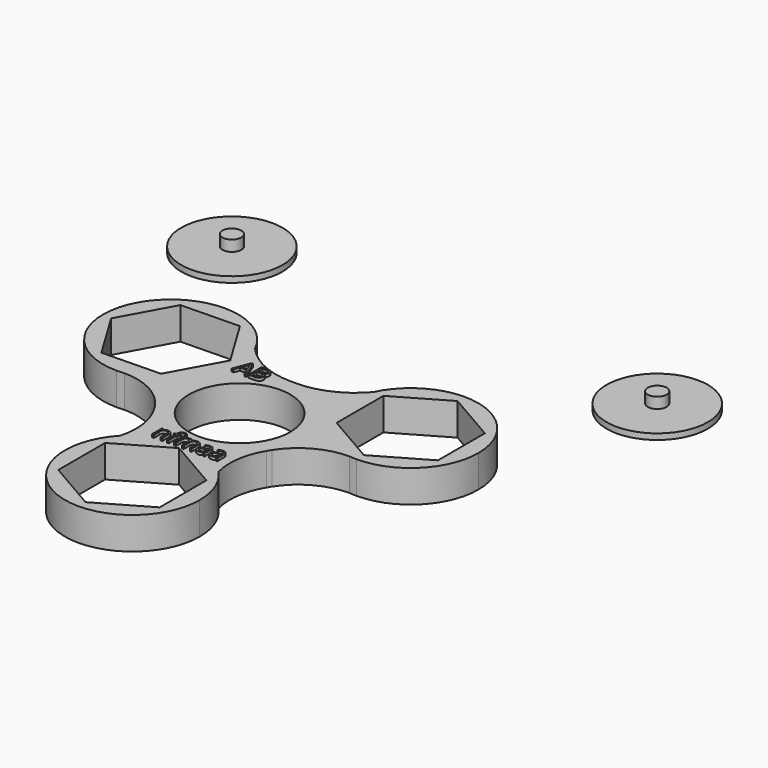
from build123d import *

# Parameters (mm, degrees)
F0_R           = 11.0297341738
F1_DEPTH       = 7.0104
F2_TEXT_SIZE   = 5.0108763389
F2_TEXT_SIZE_2 = 5.0108750454
F3_DEPTH       = 7.62
F4_R           = 2.0485624903
F5_DEPTH       = 3.6322
F4_R_2         = 11.0106906114
F6_DEPTH       = 1.27
F7_DEPTH       = 3.6322
F8_DEPTH       = 1.27


# Not quite as in the source:
# - Text() gives the source's letters only with a copy of the font that has no kerning and outlines rounded to 1/6400 em; it was checked with that copy


with BuildPart() as f1:
    # F0 (on Top) → F1 (new body)
    with BuildSketch(Plane.XY):
        with BuildLine():
            ThreePointArc((12.7688238327, -7.0845952005), (14.1366843581, -3.6590308258), (14.6025460528, 0))
            ThreePointArc((14.6025460528, 0), (10.512006113, 10.1356834356), (0.5321122622, 14.5928478292))
            ThreePointArc((0.5321122622, 14.5928478292), (0.2660161908, 14.5955055395), (0, 14.6025460528))
            ThreePointArc((0, 14.6025460528), (-0.2660161908, 14.5955055395), (-0.5321122622, 14.5928478292))
            ThreePointArc((-0.5321122622, 14.5928478292), (-12.7163913641, 7.1782826567), (-12.7688238327, -7.0845952005))
            ThreePointArc((-12.7688238327, -7.0845952005), (-12.5014299415, -7.5119719558), (-12.2495942672, -7.9486974727))
            ThreePointArc((-12.2495942672, -7.9486974727), (-7.4978531693, -12.5306244488), (-1.2139729432, -14.5519971453))
            ThreePointArc((-1.2139729432, -14.5519971453), (0, -14.50165494), (1.2139729432, -14.5519971453))
            ThreePointArc((1.2139729432, -14.5519971453), (7.4978531693, -12.5306244488), (12.2495942672, -7.9486974727))
            ThreePointArc((12.2495942672, -7.9486974727), (12.5014299415, -7.5119719558), (12.7688238327, -7.0845952005))
        make_face()
        Circle(F0_R, mode=Mode.SUBTRACT)
        with BuildLine():
            ThreePointArc((0.5321122622, 14.5928478292), (10.512006113, 10.1356834356), (14.6025460528, 0))
            ThreePointArc((14.6025460528, 0), (14.1366843581, -3.6590308258), (12.7688238327, -7.0845952005))
            ThreePointArc((12.7688238327, -7.0845952005), (17.81162254, -2.4243097964), (24.4636618418, -0.7218257358))
            ThreePointArc((24.4636618418, -0.7218257358), (13.2399010204, 6.7733722545), (12.8515015084, 20.2641078056))
            ThreePointArc((12.8515015084, 20.2641078056), (7.3157643156, 16.0730868655), (0.5321122622, 14.5928478292))
        make_face()
        with BuildLine():
            ThreePointArc((0, 14.6025460528), (0.2660161908, 14.5955055395), (0.5321122622, 14.5928478292))
            ThreePointArc((0.5321122622, 14.5928478292), (0.2661003171, 14.6001212956), (0, 14.6025460528))
        make_face()
        with BuildLine():
            ThreePointArc((12.2495942672, -7.9486974727), (12.5166680566, -7.5211283718), (12.7688238327, -7.0845952005))
            ThreePointArc((12.7688238327, -7.0845952005), (12.5014299415, -7.5119719558), (12.2495942672, -7.9486974727))
        make_face()
        with BuildLine():
            ThreePointArc((-0.5321122622, 14.5928478292), (-0.2660161908, 14.5955055395), (0, 14.6025460528))
            ThreePointArc((0, 14.6025460528), (-0.2661003171, 14.6001212956), (-0.5321122622, 14.5928478292))
        make_face()
        with BuildLine():
            ThreePointArc((40.8192647261, 13.8948662207), (29.3762925366, 28.2367891894), (12.8515015084, 20.2641078056))
            ThreePointArc((12.8515015084, 20.2641078056), (13.2399010204, 6.7733722545), (24.4636618418, -0.7218257358))
            ThreePointArc((24.4636618418, -0.7218257358), (25.2882595444, -0.7437857189), (26.1101331562, -0.8142653492))
            ThreePointArc((26.1101331562, -0.8142653492), (36.5110598346, 3.4939395422), (40.8192647261, 13.8948662207))
        make_face()
        Polygon((26.1101331562, 26.6333493906), (37.1419831871, 20.2641078056), (37.1419831871, 7.5256246357), (26.1101331562, 1.1563830507), (15.0782831253, 7.5256246357), (15.0782831253, 20.2641078056), align=None, mode=Mode.SUBTRACT)
        with BuildLine():
            ThreePointArc((10.6742573559, -19.1119285094), (10.3201713626, -13.3691904701), (12.2495942672, -7.9486974727))
            ThreePointArc((12.2495942672, -7.9486974727), (7.4978531693, -12.5306244488), (1.2139729432, -14.5519971453))
            ThreePointArc((1.2139729432, -14.5519971453), (6.3663763965, -15.9559164192), (10.6742573559, -19.1119285094))
        make_face()
        with BuildLine():
            ThreePointArc((26.1101331562, -0.8142653492), (25.2882595444, -0.7437857189), (24.4636618418, -0.7218257358))
            ThreePointArc((24.4636618418, -0.7218257358), (25.2856010357, -0.791137263), (26.1101331562, -0.8142653492))
        make_face()
        with BuildLine():
            ThreePointArc((-12.7688238327, -7.0845952005), (-12.7163913641, 7.1782826567), (-0.5321122622, 14.5928478292))
            ThreePointArc((-0.5321122622, 14.5928478292), (-7.3157643157, 16.0730868655), (-12.8515015084, 20.2641078056))
            ThreePointArc((-12.8515015084, 20.2641078056), (-11.7682101874, 17.161025601), (-11.4010015863, 13.8948662207))
            ThreePointArc((-11.4010015863, 13.8948662207), (-15.1425282506, 4.0933258226), (-24.4636618418, -0.7218257358))
            ThreePointArc((-24.4636618418, -0.7218257358), (-17.81162254, -2.4243097964), (-12.7688238327, -7.0845952005))
        make_face()
        with BuildLine():
            ThreePointArc((10.6742573559, -19.1119285094), (6.3663763965, -15.9559164192), (1.2139729432, -14.5519971453))
            ThreePointArc((1.2139729432, -14.5519971453), (0, -14.6025460528), (-1.2139729432, -14.5519971453))
            ThreePointArc((-1.2139729432, -14.5519971453), (-6.3663763965, -15.9559164192), (-10.6742573559, -19.1119285094))
            ThreePointArc((-10.6742573559, -19.1119285094), (-5.4071159221, -42.792818386), (14.6622961142, -29.1639510542))
            ThreePointArc((14.6622961142, -29.1639510542), (13.6288673318, -23.7568351321), (10.6742573559, -19.1119285094))
        make_face()
        Polygon((0, -41.889001257), (-11.02021674, -35.5264761556), (-11.02021674, -22.8014259528), (0, -16.4389008515), (11.02021674, -22.8014259528), (11.02021674, -35.5264761556), align=None, mode=Mode.SUBTRACT)
        with BuildLine():
            ThreePointArc((-12.2495942672, -7.9486974727), (-12.5014299415, -7.5119719558), (-12.7688238327, -7.0845952005))
            ThreePointArc((-12.7688238327, -7.0845952005), (-12.5166680566, -7.5211283718), (-12.2495942672, -7.9486974727))
        make_face()
        with BuildLine():
            ThreePointArc((-11.4010015863, 13.8948662207), (-11.7682101874, 17.161025601), (-12.8515015084, 20.2641078056))
            ThreePointArc((-12.8515015084, 20.2641078056), (-38.5609275889, 21.7266137608), (-26.1101331562, -0.8142653492))
            ThreePointArc((-26.1101331562, -0.8142653492), (-25.2882595444, -0.7437857189), (-24.4636618418, -0.7218257358))
            ThreePointArc((-24.4636618418, -0.7218257358), (-15.1425282506, 4.0933258226), (-11.4010015863, 13.8948662207))
        make_face()
        Polygon((-19.9787258399, 25.0606531519), (-13.3745743623, 14.1678051894), (-19.5059816786, 3.0020182582), (-32.2415404725, 2.7290792894), (-38.84569195, 13.6219272519), (-32.7142846337, 24.7877141831), align=None, mode=Mode.SUBTRACT)
        with BuildLine():
            ThreePointArc((-10.6742573559, -19.1119285094), (-6.3663763965, -15.9559164192), (-1.2139729432, -14.5519971453))
            ThreePointArc((-1.2139729432, -14.5519971453), (-7.4978531693, -12.5306244488), (-12.2495942672, -7.9486974727))
            ThreePointArc((-12.2495942672, -7.9486974727), (-10.3201713626, -13.3691904701), (-10.6742573559, -19.1119285094))
        make_face()
        with BuildLine():
            ThreePointArc((-26.1101331562, -0.8142653492), (-25.2856010357, -0.791137263), (-24.4636618418, -0.7218257358))
            ThreePointArc((-24.4636618418, -0.7218257358), (-25.2882595444, -0.7437857189), (-26.1101331562, -0.8142653492))
        make_face()
    extrude(amount=F1_DEPTH)

    # F2 (on Top) → F3 (join)
    with BuildSketch(Plane.XY):
        with Locations((-6.5103061497, -16.1879360676)):
            Text('nfmaa', F2_TEXT_SIZE, font='Open Sans', text_align=(TextAlign.LEFT, TextAlign.BOTTOM))
        with Locations((-10.5991801247, 11.1113153398)):
            Text('AB', F2_TEXT_SIZE_2, font='Open Sans', text_align=(TextAlign.LEFT, TextAlign.BOTTOM))
    extrude(amount=F3_DEPTH)


with BuildPart() as f5:
    # F4 (on Top) → F5 (new body)
    with BuildSketch(Plane.XY):
        with Locations((-46.265322715, 55.7321608067)):
            Circle(F4_R)
    extrude(amount=F5_DEPTH)

    # F4 (on Top) → F6 (join)
    with BuildSketch(Plane.XY):
        with Locations((-46.265322715, 55.7321608067)):
            Circle(F4_R_2)
        with Locations((-46.265322715, 55.7321608067)):
            Circle(F4_R, mode=Mode.SUBTRACT)
    extrude(amount=F6_DEPTH)


with BuildPart() as f7:
    # F4 (on Top) → F7 (new body)
    with BuildSketch(Plane.XY):
        with Locations((46.265322715, 55.7321608067)):
            Circle(F4_R)
    extrude(amount=F7_DEPTH)

    # F4 (on Top) → F8 (join)
    with BuildSketch(Plane.XY):
        with Locations((46.265322715, 55.7321608067)):
            Circle(F4_R_2)
        with Locations((46.265322715, 55.7321608067)):
            Circle(F4_R, mode=Mode.SUBTRACT)
    extrude(amount=F8_DEPTH)


solid = Compound([f1.part, f5.part, f7.part])
